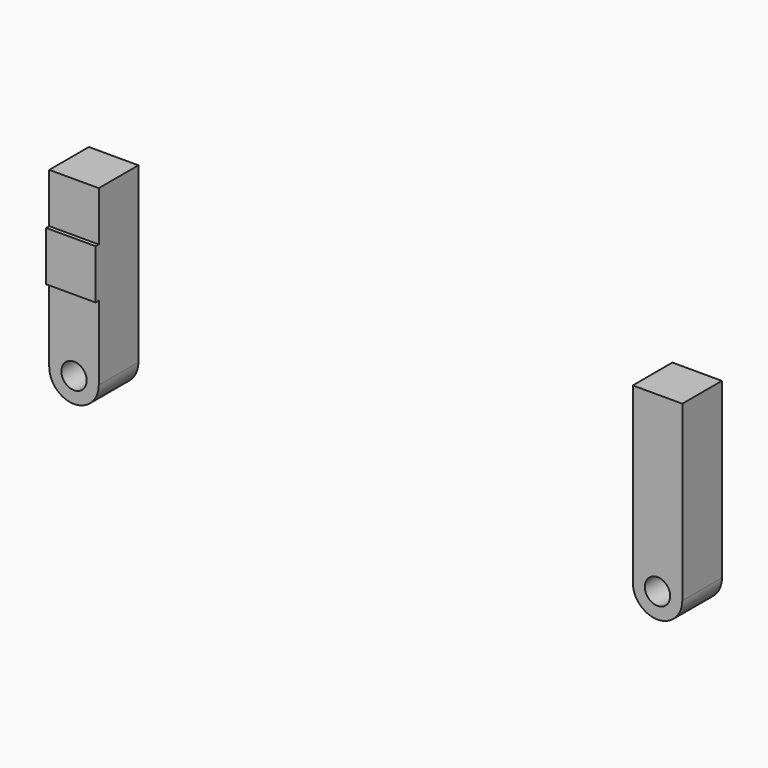
from build123d import *

# Parameters (mm, degrees)
F0_W     = 3.175
F0_H     = 12.7
F0_R     = 0.8128
F1_DEPTH = 1.5875
F2_R     = 1.58749
F4_W     = 3.175
F4_H     = 3.175
F5_DEPTH = 0.254


# Not quite as in the source:
# - a fillet or chamfer is up to 0.001 mm smaller than in the source, because OpenCascade refuses the exact size


with BuildPart() as f1:
    # F0 (on Front) → F1 (new body, symmetric)
    with BuildSketch(Plane.XZ):
        with Locations((-18.7037093565, 0.3757816428)):
            Rectangle(F0_W, F0_H)
        with Locations((-18.7037093565, -4.3867183572)):
            Circle(F0_R, mode=Mode.SUBTRACT)
    extrude(amount=F1_DEPTH, both=True)

    # F2 (radius 1.5875 in the source; OpenCascade refuses exactly that, so slightly less here)
    f2_edges = [f1.edges().sort_by_distance(p)[0] for p in [
        (-20.291209, 0, -5.974218),
        (-17.116209, 0, -5.974218),
    ]]
    fillet(f2_edges, radius=F2_R)


with BuildPart() as f3_1:
    # F3: instance of F1
    add(f1.part.mirror(Plane.YZ))


with BuildPart() as f1_1:
    add(f1.part)

    # F4 (on face) → F5 (join)
    with BuildSketch(Plane.XZ.offset(1.5875)):
        with Locations((-18.7037093565, 1.9632816428)):
            Rectangle(F4_W, F4_H)
    extrude(amount=F5_DEPTH)


solid = Compound([f3_1.part, f1_1.part])
